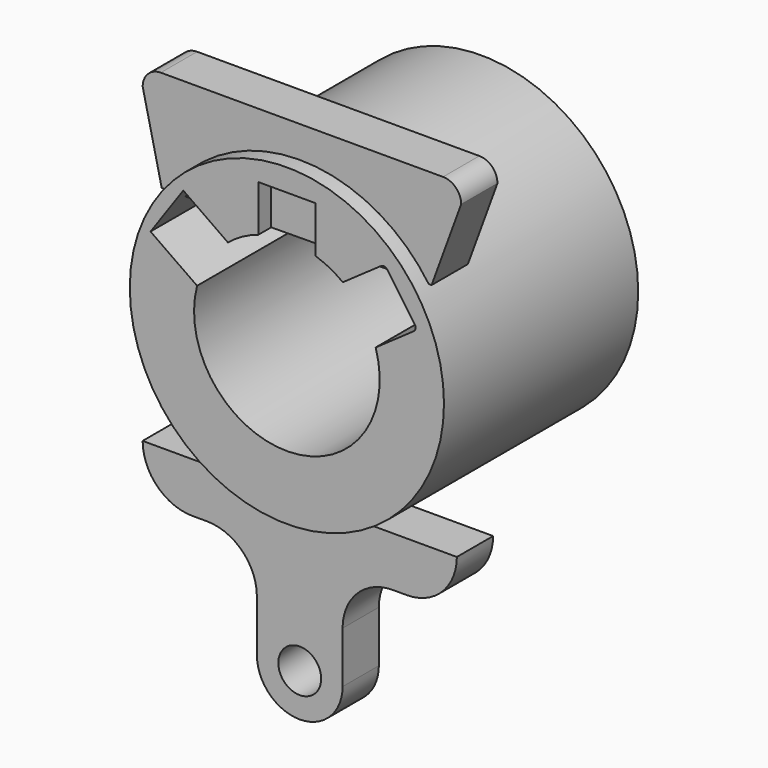
from build123d import *

# Parameters (mm, degrees)
F0_R      = 44
F1_DEPTH  = 68
F7_DEPTH  = 68.001
F10_DEPTH = 12.7
F13_DEPTH = 12.7
F14_DEPTH = 12.7
F17_DEPTH = 12.7


# Not quite as in the source:
# - a feature names something its author has since deleted; it is built from what else it names


with BuildPart() as f1:
    # F0 (on Front) → F1 (new body)
    with BuildSketch(Plane.XZ):
        Circle(F0_R)
    extrude(amount=F1_DEPTH)

    # F3 (on offset) → F7 (cut, through all)
    with BuildSketch(Plane.XZ.offset(68)):
        with BuildLine():
            Line((26.3302369395, 28.2014110136), (15.6770635175, 20.7419786777))
            ThreePointArc((15.6770635175, 20.7419786777), (12.0064707427, 23.0617575285), (8.001, 24.7383103505))
            ThreePointArc((8.001, 24.7383103505), (0.0005254973, 25.9999999947), (-8, 24.7386337537))
            ThreePointArc((-8, 24.7386337537), (-12.480459792, 22.8087291049), (-16.5215362846, 20.0758272257))
            Line((-16.5215362846, 20.0758272257), (-29.0134122429, 28.8227329381))
            Line((-29.0134122429, 28.8227329381), (-38.1906352245, 15.7163002295))
            Line((-38.1906352245, 15.7163002295), (-25.15190359, 6.5864820503))
            ThreePointArc((-25.15190359, 6.5864820503), (0.5451088298, -25.9942850712), (24.8536719418, 7.6351156514))
            Line((24.8536719418, 7.6351156514), (35.5074599211, 15.094978305))
            ThreePointArc((35.5074599211, 15.094978305), (36.0297236932, 15.9147682156), (35.8193409432, 16.8637434754))
            Line((35.8193409432, 16.8637434754), (28.0990021099, 27.8895299915))
            ThreePointArc((28.0990021099, 27.8895299915), (27.2792121993, 28.4117937637), (26.3302369395, 28.2014110136))
        make_face()
        with BuildLine():
            ThreePointArc((-8, 24.7386337537), (0.0005254973, 25.9999999947), (8.001, 24.7383103505))
            Line((8.001, 24.7383103505), (8.001, 37.7434337537))
            Line((8.001, 37.7434337537), (0, 37.7434337537))
            Line((0, 37.7434337537), (-8, 37.7434337537))
            Line((-8, 37.7434337537), (-8, 24.7386337537))
        make_face()
    extrude(amount=-F7_DEPTH, mode=Mode.SUBTRACT)

    # F6 (on offset) → F14 (join)
    with BuildSketch(Plane.XZ.offset(50.8)):
        with BuildLine():
            Line((44.0054678571, -39.6192881453), (0, -39.6192881453))
            Line((0, -39.6192881453), (-44.0054678571, -39.6192881453))
            ThreePointArc((-44.0054678571, -39.6192881453), (-39.8943826467, -49.4993840076), (-30.0055, -53.5892881453))
            Line((-30.0055, -53.5892881453), (-26, -53.5892881453))
            ThreePointArc((-26, -53.5892881453), (-16.1005050634, -57.6897932087), (-12, -67.5892881453))
            Line((-12, -67.5892881453), (-12, -82))
            ThreePointArc((-12, -82), (-8.4852813742, -90.4852813742), (0, -94))
            ThreePointArc((0, -94), (8.4852813742, -90.4852813742), (12, -82))
            Line((12, -82), (12, -67.5892881453))
            ThreePointArc((12, -67.5892881453), (16.1005050634, -57.6897932087), (26, -53.5892881453))
            Line((26, -53.5892881453), (30.0055, -53.5892881453))
            ThreePointArc((30.0055, -53.5892881453), (39.8943826467, -49.4993840076), (44.0054678571, -39.6192881453))
        make_face()
        with BuildLine():
            ThreePointArc((6, -82), (-4.2426406871, -86.2426406871), (0, -76))
            ThreePointArc((0, -76), (4.2426406871, -77.7573593129), (6, -82))
        make_face(mode=Mode.SUBTRACT)
    extrude(amount=F14_DEPTH)

    # F16 (on offset) → F17 (join)
    with BuildSketch(Plane.XZ.offset(50.8)):
        with BuildLine():
            ThreePointArc((45.2163087713, 47.7545370714), (43.7284112197, 51.3466395198), (40.1363087713, 52.8345370714))
            Line((40.1363087713, 52.8345370714), (-38.9128, 52.8345370714))
            ThreePointArc((-38.9128, 52.8345370714), (-42.5049024484, 51.3466395198), (-43.9928, 47.7545370714))
            Line((-43.9928, 47.7545370714), (-38.6563204229, 24.4916565716))
            Line((-38.6563204229, 24.4916565716), (36.9281843305, 25.1138713211))
            Line((36.9281843305, 25.1138713211), (45.2163087713, 47.7545370714))
        make_face()
    extrude(amount=F17_DEPTH)


with BuildPart() as f10:
    # F9 (on face) → F10 (new body)
    with BuildSketch(Plane(origin=(0, 0, 0), x_dir=(0, -1, 0), z_dir=(-0.8191520443, 0, 0.5735764364))):
        Polygon((-12.0716131376, -17.2400502406), (0, 0), (-12.0716131376, 0), align=None)
    extrude(amount=F10_DEPTH)

    # F12 (on face) → F13 (join)
    with BuildSketch(Plane(origin=(0, 0, 0), x_dir=(0, -1, 0), z_dir=(-0.9396926208, 0, -0.3420201433))):
        Polygon((0, 0), (-13.8556587323, 0), (-14.1112022102, -13.5903209448), align=None)
    extrude(amount=F13_DEPTH)


solid = Compound([f1.part, f10.part])
